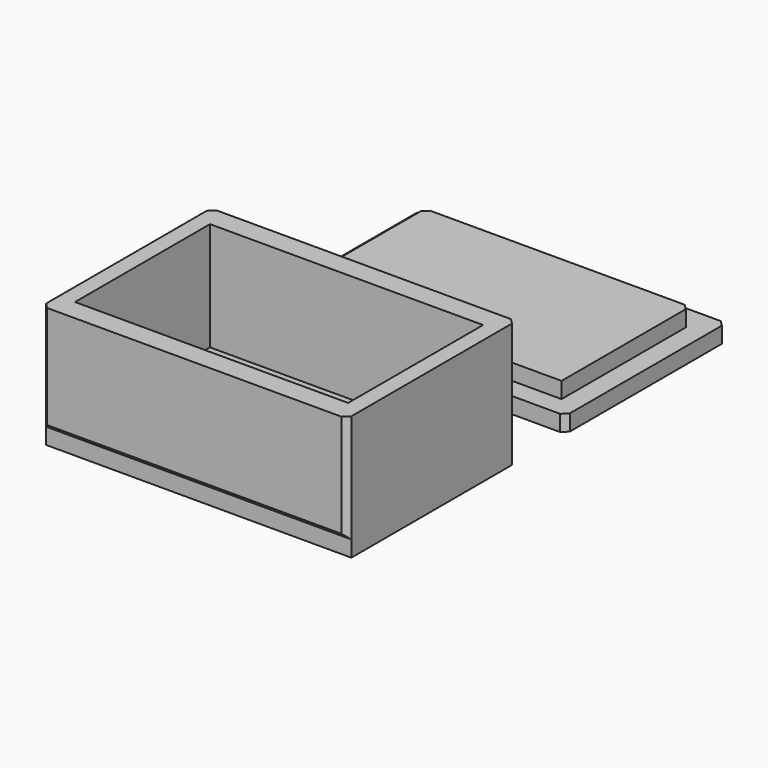
from build123d import *

# Parameters (mm, degrees)
F0_W      = 22.8
F0_H      = 15
F1_DEPTH  = 1.2
F2_W      = 22.8
F2_H      = 0.4
F2_H_2    = 15
F2_W_2    = 20.4
F2_H_3    = 12.6
F3_DEPTH  = 8.1
F4_W      = 19.8
F4_H      = 12
F5_DEPTH  = 1.2
F6_SIZE   = 0.39999
F6_2_SIZE = 0.39999


# Not quite as in the source:
# - a fillet or chamfer is up to 0.001 mm smaller than in the source, because OpenCascade refuses the exact size


with BuildPart() as f1:
    # F0 (on Top) → F1 (new body)
    with BuildSketch(Plane.XY):
        Rectangle(F0_W, F0_H)
    extrude(amount=F1_DEPTH)

    # F2 (on face) → F3 (join)
    with BuildSketch(Plane.XY.offset(1.2)):
        with Locations((0, 7.7)):
            Rectangle(F2_W, F2_H)
        Rectangle(F2_W, F2_H_2)
        Rectangle(F2_W_2, F2_H_3, mode=Mode.SUBTRACT)
        with Locations((0, -7.7)):
            Rectangle(F2_W, F2_H)
    extrude(amount=F3_DEPTH)

    # F6 (size 0.4 in the source; OpenCascade refuses exactly that, so slightly less here)
    f6_edges = [f1.edges().sort_by_distance(p)[0] for p in [
        (0, -7.9, 1.2),
        (11.4, -7.9, 5.25),
        (-11.4, -7.9, 5.25),
        (11.4, 7.9, 5.25),
        (0, 7.9, 1.2),
        (-11.4, 7.9, 5.25),
    ]]
    chamfer(f6_edges, length=F6_SIZE)


with BuildPart() as f1b:
    # F0 (on Top) → F1, piece 2 (new body)
    with BuildSketch(Plane.XY):
        with Locations((0, 20)):
            Rectangle(F0_W, F0_H)
    extrude(amount=F1_DEPTH)

    # F4 (on face) → F5 (join)
    with BuildSketch(Plane.XY.offset(1.2)):
        with Locations((0, 20)):
            Rectangle(F4_W, F4_H)
    extrude(amount=F5_DEPTH)

    # F6#2 (size 0.4 in the source; OpenCascade refuses exactly that, so slightly less here)
    f6_2_edges = [f1b.edges().sort_by_distance(p)[0] for p in [
        (11.4, 12.5, 0.6),
        (-11.4, 12.5, 0.6),
        (-11.4, 27.5, 0.6),
        (-9.9, 26, 1.8),
        (-9.9, 14, 1.8),
        (11.4, 27.5, 0.6),
        (9.9, 26, 1.8),
    ]]
    chamfer(f6_2_edges, length=F6_2_SIZE)


solid = Compound([f1.part, f1b.part])
